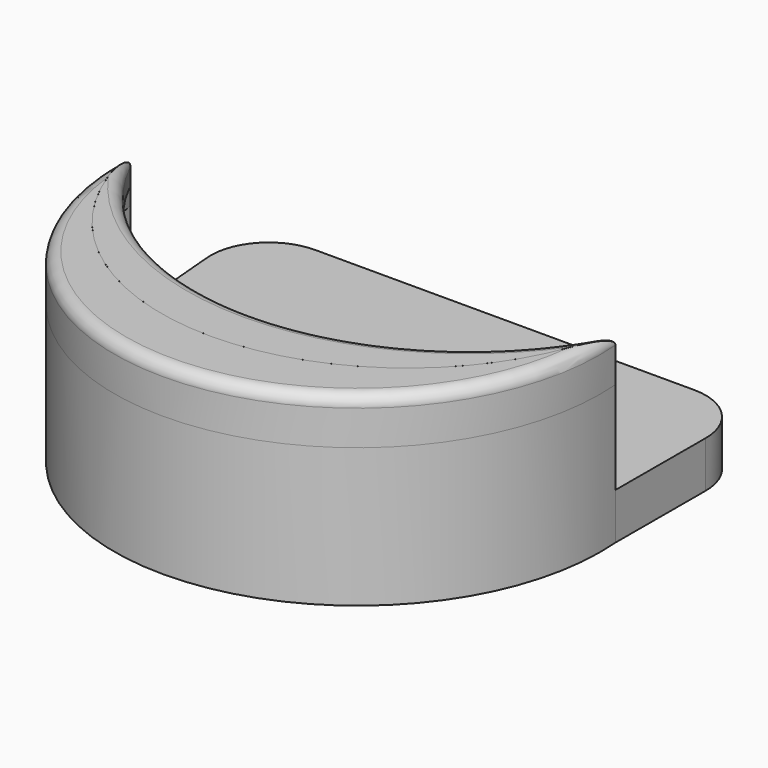
from build123d import *

# Parameters (mm, degrees)
F0_R        = 3
F1_DEPTH    = 4
F2_DEPTH    = 12
F3_START    = 12
F3_DEPTH    = 4
F4_R        = 5
F5_START    = 13.5
F5_DEPTH    = 2.5
F6_T2_ANGLE = 202.7002250933
F7_R        = 1
F8_SIZE     = 1.5


# Not quite as in the source:
# - a fillet or chamfer that OpenCascade refuses, or shapes differently, is made with other operations: its cross-section is extruded or revolved along the edge and cut away or added


with BuildPart() as f1:
    # F0 (on Top) → F1 (new body)
    with BuildSketch(Plane.XY):
        with BuildLine():
            Line((-43.1358516216, 14.7124025971), (-41.8695434246, 0))
            ThreePointArc((-41.8695434246, 0), (-20.9347717123, -12.9699445096), (0, 0))
            Line((0, 0), (0.0331684333, 14.7124025971))
            Line((0.0331684333, 14.7124025971), (-43.1358516216, 14.7124025971))
        make_face()
        with Locations((-20.9347717123, 0.0471964775)):
            Circle(F0_R, mode=Mode.SUBTRACT)
        with BuildLine():
            ThreePointArc((0, 0), (-20.9347717123, -20.8876284359), (-41.8695434246, 0))
            ThreePointArc((-41.8695434246, 0), (-20.9347717123, -22.6538843228), (0, 0))
        make_face()
        with BuildLine():
            ThreePointArc((0, 0), (-20.9347717123, -17.5236648917), (-41.8695434246, 0))
            ThreePointArc((-41.8695434246, 0), (-20.9347717123, -20.8876284359), (0, 0))
        make_face()
        with BuildLine():
            ThreePointArc((0, 0), (-20.9347717123, -12.9699445096), (-41.8695434246, 0))
            ThreePointArc((-41.8695434246, 0), (-20.9347717123, -17.5236648917), (0, 0))
        make_face()
    extrude(amount=F1_DEPTH)

    # F0 (on Top) → F2 (join)
    with BuildSketch(Plane.XY):
        with BuildLine():
            ThreePointArc((0, 0), (-20.9347717123, -20.8876284359), (-41.8695434246, 0))
            ThreePointArc((-41.8695434246, 0), (-20.9347717123, -22.6538843228), (0, 0))
        make_face()
    extrude(amount=F2_DEPTH)

    # F4
    f4_edges = [f1.edges().sort_by_distance(p)[0] for p in [
        (0.033168, 14.712403, 2),
        (-43.135852, 14.712403, 2),
    ]]
    fillet(f4_edges, radius=F4_R)

    # F8
    f8_edges = [f1.edges().sort_by_distance(p)[0] for p in [
        (-23.934772, 0.047196, 4),
    ]]
    chamfer(f8_edges, length=F8_SIZE)


with BuildPart() as f3:
    # F0 (on Top) → F3 (new body)
    with BuildSketch(Plane.XY.offset(F3_START)):
        with BuildLine():
            ThreePointArc((0, 0), (-20.9347717123, -17.5236648917), (-41.8695434246, 0))
            ThreePointArc((-41.8695434246, 0), (-20.9347717123, -20.8876284359), (0, 0))
        make_face()
        with BuildLine():
            ThreePointArc((0, 0), (-20.9347717123, -20.8876284359), (-41.8695434246, 0))
            ThreePointArc((-41.8695434246, 0), (-20.9347717123, -22.6538843228), (0, 0))
        make_face()
    extrude(amount=F3_DEPTH)

    # F6: fillet of radius 1 on 1 edges, made by hand

    # F6_s1 → F6_t2 (revolve, cut)
    with BuildSketch(Plane(origin=(-1.1299645501, -5.6292919355, 0), x_dir=(0, 0, 1), z_dir=(0.1968037431, 0.9804429033, 0))):
        with BuildLine():
            ThreePointArc((15, -41.1998577327), (15.7071067812, -40.9069645139), (16, -40.1998577327))
            Line((16, -40.1998577327), (16, -41.1998577327))
            Line((16, -41.1998577327), (15, -41.1998577327))
        make_face()
    revolve(axis=Axis((-20.9347717123, -1.6538843228, 16), (0, 0, 1)), revolution_arc=F6_T2_ANGLE, mode=Mode.SUBTRACT)


with BuildPart() as f5:
    # F0 (on Top) → F5 (new body)
    with BuildSketch(Plane.XY.offset(F5_START)):
        with BuildLine():
            ThreePointArc((0, 0), (-20.9347717123, -12.9699445096), (-41.8695434246, 0))
            ThreePointArc((-41.8695434246, 0), (-20.9347717123, -17.5236648917), (0, 0))
        make_face()
    extrude(amount=F5_DEPTH)

    # F7
    f7_edges = [f5.edges().sort_by_distance(p)[0] for p in [
        (-20.934772, -12.969945, 16),
    ]]
    fillet(f7_edges, radius=F7_R)


solid = Compound([f1.part, f3.part, f5.part])
